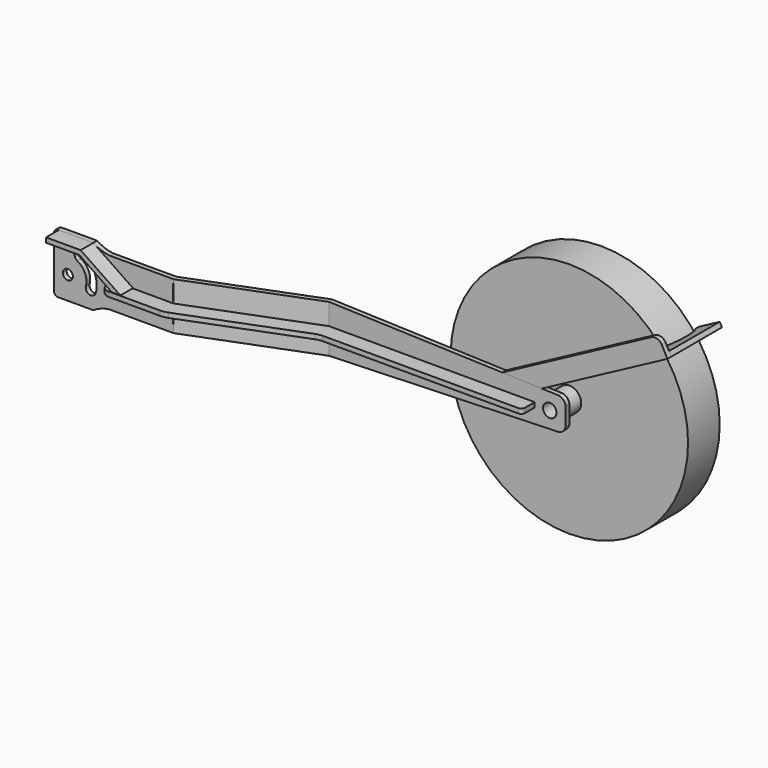
from build123d import *

# Parameters (mm, degrees)
F1_DEPTH  = 60
F3_R      = 8.25
F4_DEPTH  = 25
F5_DEPTH  = 6
F6_R      = 6.375
F7_DEPTH  = 25
F10_DEPTH = 6
F11_DEPTH = 6
F12_DEPTH = 25
F13_DEPTH = 25
F14_W     = 1
F14_H     = 20
F14_H_2   = 15
F15_DEPTH = 25
F17_DEPTH = 20
F18_R     = 15
F19_DEPTH = 25
F21_DEPTH = 50
F23_DEPTH = 6
F25_DEPTH = 80
F27_DEPTH = 25
F28_R     = 8.5
F29_DEPTH = 86.001


# Not quite as in the source:
# - a feature names something its author has since deleted; it is built from what else it names


with BuildPart() as f1:
    # F0 (on Top) → F1 (new body)
    with BuildSketch(Plane.XY):
        Polygon((-150, 0), (-300, 0), (-300, -6), (-148.8803913162, -6), (1.1196086838, 52), (300.12, 52), (300, 58), (0, 58), align=None)
    extrude(amount=F1_DEPTH)

    # F3 (on face) → F4 (cut)
    with BuildSketch(Plane.XZ.offset(-52)):
        with BuildLine():
            Line((300.12, 60), (1.1196086838, 60))
            Line((1.1196086838, 60), (290.4542608309, 50.3232684455))
            ThreePointArc((290.4542608309, 50.3232684455), (297.3082754646, 47.2807408597), (300.12, 40.3288565219))
            Line((300.12, 40.3288565219), (300.12, 60))
        make_face()
        with BuildLine():
            Line((290.4542608309, 9.6767315545), (1.1196086838, 0))
            Line((1.1196086838, 0), (300.12, 0))
            Line((300.12, 0), (300.12, 19.6711434781))
            ThreePointArc((300.12, 19.6711434781), (297.3082754646, 12.7192591403), (290.4542608309, 9.6767315545))
        make_face()
        with Locations((280.12, 30.0079316213)):
            Circle(F3_R)
    extrude(amount=-F4_DEPTH, mode=Mode.SUBTRACT)

    # F2 (on face) → F5 (join)
    with BuildSketch(Plane.XZ.offset(6)):
        with BuildLine():
            Line((-250.3, 67.5), (-295, 67.5))
            ThreePointArc((-295, 67.5), (-298.5355339059, 66.0355339059), (-300, 62.5))
            Line((-300, 62.5), (-300, 60))
            Line((-300, 60), (-230, 60))
            ThreePointArc((-230, 60), (-240.6075702178, 62.5115099439), (-250.3, 67.5))
        make_face()
    extrude(amount=-F5_DEPTH)

    # F6 (on face) → F7 (cut)
    with BuildSketch(Plane.XZ.offset(6)):
        with BuildLine():
            ThreePointArc((-259.7213383401, 16.1343621796), (-255.0196238496, 8.2353824448), (-247.1206441149, 12.9370969353))
            ThreePointArc((-247.1206441149, 12.9370969353), (-248.9955051627, 35.6089750865), (-264.4106548881, 52.339256668))
            ThreePointArc((-264.4106548881, 52.339256668), (-273.2189113282, 49.7096904517), (-270.5893451119, 40.9014340116))
            ThreePointArc((-270.5893451119, 40.9014340116), (-260.8998224273, 30.3852570175), (-259.7213383401, 16.1343621796))
        make_face()
        with Locations((-282.545583065, 21.5497146659)):
            Circle(F6_R)
    extrude(amount=-F7_DEPTH, mode=Mode.SUBTRACT)

    # F2 (on face) → F11 (join)
    with BuildSketch(Plane.XZ.offset(6)):
        with BuildLine():
            Line((-250.3, 67.5), (-295, 67.5))
            ThreePointArc((-295, 67.5), (-298.5355339059, 66.0355339059), (-300, 62.5))
            Line((-300, 62.5), (-300, 60))
            Line((-300, 60), (-300, 0))
            Line((-300, 0), (-300, -2.5))
            ThreePointArc((-300, -2.5), (-298.5355339059, -6.0355339059), (-295, -7.5))
            Line((-295, -7.5), (-250.3, -7.5))
            ThreePointArc((-250.3, -7.5), (-240.6075702178, -2.5115099439), (-230, 0))
            Line((-230, 0), (-230, 60))
            ThreePointArc((-230, 60), (-240.6075702178, 62.5115099439), (-250.3, 67.5))
        make_face()
    extrude(amount=-F11_DEPTH)

    # F6 (on face) → F12 (cut)
    with BuildSketch(Plane.XZ.offset(6)):
        with BuildLine():
            ThreePointArc((-259.7213383401, 16.1343621796), (-255.0196238496, 8.2353824448), (-247.1206441149, 12.9370969353))
            ThreePointArc((-247.1206441149, 12.9370969353), (-248.9955051627, 35.6089750865), (-264.4106548881, 52.339256668))
            ThreePointArc((-264.4106548881, 52.339256668), (-273.2189113282, 49.7096904517), (-270.5893451119, 40.9014340116))
            ThreePointArc((-270.5893451119, 40.9014340116), (-260.8998224273, 30.3852570175), (-259.7213383401, 16.1343621796))
        make_face()
        with Locations((-282.545583065, 21.5497146659)):
            Circle(F6_R)
    extrude(amount=-F12_DEPTH, mode=Mode.SUBTRACT)

    # F6 (on face) → F13 (cut)
    with BuildSketch(Plane.XZ.offset(6)):
        with BuildLine():
            ThreePointArc((-259.7213383401, 16.1343621796), (-255.0196238496, 8.2353824448), (-247.1206441149, 12.9370969353))
            ThreePointArc((-247.1206441149, 12.9370969353), (-248.9955051627, 35.6089750865), (-264.4106548881, 52.339256668))
            ThreePointArc((-264.4106548881, 52.339256668), (-273.2189113282, 49.7096904517), (-270.5893451119, 40.9014340116))
            ThreePointArc((-270.5893451119, 40.9014340116), (-260.8998224273, 30.3852570175), (-259.7213383401, 16.1343621796))
        make_face()
        with Locations((-282.545583065, 21.5497146659)):
            Circle(F6_R)
    extrude(amount=-F13_DEPTH, mode=Mode.SUBTRACT)

    # F14 (on face) → F15 (cut)
    with BuildSketch(Plane.XZ.offset(6)):
        with Locations((-149.3803913162, 45)):
            Rectangle(F14_W, F14_H)
        with Locations((-149.3803913162, 17.5)):
            Rectangle(F14_W, F14_H_2)
    extrude(amount=-F15_DEPTH, mode=Mode.SUBTRACT)

    # F18 (on face) → F19 (join)
    with BuildSketch(Plane(origin=(0, 58, 0), x_dir=(-1, 0, 0), z_dir=(0, 1, 0))):
        with Locations((-280.12, 30.0079316213)):
            Circle(F18_R)
    extrude(amount=F19_DEPTH)

    # F20 (on face) → F21 (join)
    with BuildSketch(Plane(origin=(0, 83, 0), x_dir=(-1, 0, 0), z_dir=(0, 1, 0))):
        with BuildLine():
            ThreePointArc((-306.8151369112, 177.6133843163), (-376.2858189362, -85.1099873502), (-130.12, 30.0079316213))
            ThreePointArc((-130.12, 30.0079316213), (-183.9541810638, 145.1258505929), (-306.8151369112, 177.6133843163))
        make_face()
    extrude(amount=F21_DEPTH)

    # F28 (on face) → F29 (cut, through all)
    with BuildSketch(Plane.XZ.offset(-52)):
        with Locations((280.12, 30.0079316213)):
            Circle(F28_R)
    extrude(amount=-F29_DEPTH, mode=Mode.SUBTRACT)


with BuildPart() as f10:
    # F9 (on offset) → F10 (new body)
    with BuildSketch(Plane(origin=(0, 0, 33), x_dir=(1, 0, 0), z_dir=(0, 0, -1))):
        with BuildLine():
            Line((-225.14836237, 16), (-225.14836237, 6))
            Line((-225.14836237, 6), (-148.8803913162, 6))
            Line((-148.8803913162, 6), (1.1196086838, -52))
            Line((1.1196086838, -52), (261.1196086838, -52))
            Line((261.1196086838, -52), (261.1196086838, -37))
            ThreePointArc((261.1196086838, -37), (259.6551425898, -33.4644660941), (256.1196086838, -32))
            Line((256.1196086838, -32), (9.5166738126, -32))
            ThreePointArc((9.5166738126, -32), (4.930794843, -31.5757952888), (0.5005439906, -30.3175771261))
            Line((0.5005439906, -30.3175771261), (-140.7972687306, 24.3175771261))
            ThreePointArc((-140.7972687306, 24.3175771261), (-145.2275195831, 25.5757952888), (-149.8133985527, 26))
            Line((-149.8133985527, 26), (-215.14836237, 26))
            ThreePointArc((-215.14836237, 26), (-222.2194301819, 23.0710678119), (-225.14836237, 16))
        make_face()
    extrude(amount=F10_DEPTH)


with BuildPart() as f17:
    # F16 (on face) → F17 (new body)
    with BuildSketch(Plane.XZ.offset(6)):
        Polygon((-250.3, 67.5), (-294.0215170383, 67.5), (-294.0215170383, 61.5), (-252.1453078549, 61.5), (-210.7984625637, 33.4105253768), (-200.1213386967, 33.4105253768), align=None)
    extrude(amount=F17_DEPTH)


with BuildPart() as f23:
    # F22 (on face) → F23 (new body)
    with BuildSketch(Plane.XZ.offset(-52)):
        with BuildLine():
            Line((270.12, 51.0033431685), (428.9258106677, 135.7424398015))
            Line((428.9258106677, 135.7424398015), (421.8642192816, 148.9762573572))
            ThreePointArc((421.8642192816, 148.9762573572), (415.9512895642, 153.8358772929), (408.3339466538, 153.0910748035))
            Line((408.3339466538, 153.0910748035), (220.1479403824, 52.6746473229))
            Line((220.1479403824, 52.6746473229), (270.12, 51.0033431685))
        make_face()
    extrude(amount=-F23_DEPTH)


with BuildPart() as f25:
    # F24 (on face) → F25 (new body)
    with BuildSketch(Plane(origin=(0, 58, 0), x_dir=(-1, 0, 0), z_dir=(0, 1, 0))):
        Polygon((-426.1011741132, 141.0359668238), (-428.9258106677, 135.7424398015), (-402.4581755564, 121.6192570294), (-399.633539002, 126.9127840516), align=None)
    extrude(amount=F25_DEPTH)

    # F26 (on face) → F27 (cut)
    with BuildSketch(Plane(origin=(35.8574468804, 0, -67.1988627041), x_dir=(0.8822545037, 0, 0.4707727591), z_dir=(-0.4707727591, 0, 0.8822545037))):
        with BuildLine():
            Line((412.3255711273, 133), (412.3255711273, 83))
            ThreePointArc((412.3255711273, 83), (422.3255711273, 108), (412.3255711273, 133))
        make_face()
    extrude(amount=-F27_DEPTH, mode=Mode.SUBTRACT)


solid = Compound([f1.part, f10.part, f17.part, f23.part, f25.part])
